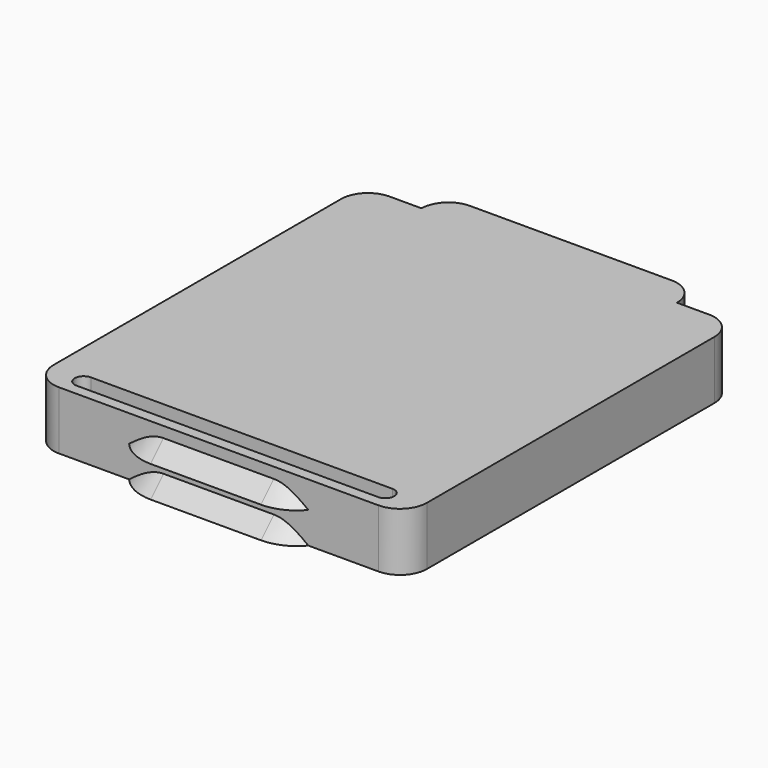
from build123d import *

# Parameters (mm, degrees)
F0_W        = 41.65
F0_H        = 46.1
F1_DEPTH    = 6.5
F2_W        = 28.5
F2_H        = 3
F3_DEPTH    = 3
F4_R        = 1
F5_T1_DEPTH = 10.5
F5_T4_ANGLE = 90
F5_T6_ANGLE = 90
F6_W        = 20
F6_H        = 1.8
F7_DEPTH    = 1.8
F8_T1_DEPTH = 21.0093727123
F8_T3_DEPTH = 21.0093727123
F9_SIZE2    = 1.79999
F9_SIZE     = 1.79999
F10_R       = 3


# Not quite as in the source:
# - a fillet or chamfer that OpenCascade refuses, or shapes differently, is made with other operations: its cross-section is extruded or revolved along the edge and cut away or added
# - a fillet or chamfer is up to 0.001 mm smaller than in the source, because OpenCascade refuses the exact size


with BuildPart() as f1:
    # F0 (on Top) → F1 (new body)
    with BuildSketch(Plane.XY):
        Rectangle(F0_W, F0_H)
        with BuildLine():
            ThreePointArc((16.825, -19.85), (17.825, -20.85), (16.825, -21.85))
            Line((16.825, -21.85), (-16.825, -21.85))
            ThreePointArc((-16.825, -21.85), (-17.825, -20.85), (-16.825, -19.85))
            Line((-16.825, -19.85), (16.825, -19.85))
        make_face(mode=Mode.SUBTRACT)
    extrude(amount=F1_DEPTH)

    # F2 (on face) → F3 (join)
    with BuildSketch(Plane(origin=(0, 23.05, 0), x_dir=(-1, 0, 0), z_dir=(0, 1, 0))):
        with Locations((0, 5)):
            Rectangle(F2_W, F2_H)
    extrude(amount=F3_DEPTH)

    # F4
    f4_edges = [f1.edges().sort_by_distance(p)[0] for p in [
        (-14.25, 24.55, 3.5),
        (14.25, 24.55, 3.5),
        (0, 26.05, 3.5),
    ]]
    fillet(f4_edges, radius=F4_R)

    # F5: fillet of radius 3 on 3 edges, made by hand

    # F5_s2 → F5_t1 (cut)
    with BuildSketch(Plane.XY.offset(3.5)):
        with BuildLine():
            ThreePointArc((14.25, 23.05), (13.3713203436, 25.1713203436), (11.25, 26.05))
            Line((11.25, 26.05), (14.25, 26.05))
            Line((14.25, 26.05), (14.25, 23.05))
        make_face()
        with BuildLine():
            ThreePointArc((-14.25, 23.05), (-13.3713203436, 25.1713203436), (-11.25, 26.05))
            Line((-11.25, 26.05), (-14.25, 26.05))
            Line((-14.25, 26.05), (-14.25, 23.05))
        make_face()
    extrude(amount=F5_T1_DEPTH, mode=Mode.SUBTRACT)

    # F5_s3 → F5_t4 (revolve, cut)
    with BuildSketch(Plane.XZ.offset(-23.05)):
        with BuildLine():
            ThreePointArc((-13.25, 3.5), (-13.9571067812, 3.7928932188), (-14.25, 4.5))
            Line((-14.25, 4.5), (-14.25, 3.5))
            Line((-14.25, 3.5), (-13.25, 3.5))
        make_face()
    revolve(axis=Axis((-11.25, 23.05, 3.5), (0, 0, -1)), revolution_arc=F5_T4_ANGLE, mode=Mode.SUBTRACT)

    # F5_s5 → F5_t6 (revolve, cut)
    with BuildSketch(Plane.YZ.offset(11.25)):
        with BuildLine():
            ThreePointArc((25.05, 3.5), (25.7571067812, 3.7928932188), (26.05, 4.5))
            Line((26.05, 4.5), (26.05, 3.5))
            Line((26.05, 3.5), (25.05, 3.5))
        make_face()
    revolve(axis=Axis((11.25, 23.05, 3.5), (0, 0, -1)), revolution_arc=F5_T6_ANGLE, mode=Mode.SUBTRACT)

    # F6 (on face) → F7 (join)
    with BuildSketch(Plane.XZ.offset(23.05)):
        with Locations((0, 4.4)):
            Rectangle(F6_W, F6_H)
        with Locations((0, 0.9)):
            Rectangle(F6_W, F6_H)
    extrude(amount=F7_DEPTH)

    # F8: fillet of radius 5 on 4 edges, made by hand

    # F8_s2 → F8_t1 (cut)
    with BuildSketch(Plane.XY.offset(-6.1046863561)):
        with BuildLine():
            ThreePointArc((-10, -23.05), (-8.2794458011, -24.3776925691), (-6.1581254575, -24.85))
            Line((-6.1581254575, -24.85), (-6.1581254575, -24.95))
            Line((-6.1581254575, -24.95), (-10, -24.95))
            Line((-10, -24.95), (-10.1, -24.85))
            ThreePointArc((-10.1, -24.85), (-10.1, -23.95), (-10.0768374908, -23.114))
            Line((-10.0768374908, -23.114), (-10, -23.05))
        make_face()
        with BuildLine():
            ThreePointArc((10, -23.05), (8.2794458011, -24.3776925691), (6.1581254575, -24.85))
            Line((6.1581254575, -24.85), (6.1581254575, -24.95))
            Line((6.1581254575, -24.95), (10, -24.95))
            Line((10, -24.95), (10.1, -24.85))
            ThreePointArc((10.1, -24.85), (10.1, -23.95), (10.0768374908, -23.114))
            Line((10.0768374908, -23.114), (10, -23.05))
        make_face()
    extrude(amount=F8_T1_DEPTH, mode=Mode.SUBTRACT)

    # F8_s4 → F8_t3 (cut)
    with BuildSketch(Plane.XY.offset(-9.6046863561)):
        with BuildLine():
            ThreePointArc((-10, -23.05), (-8.2794458011, -24.3776925691), (-6.1581254575, -24.85))
            Line((-6.1581254575, -24.85), (-6.1581254575, -24.95))
            Line((-6.1581254575, -24.95), (-10, -24.95))
            Line((-10, -24.95), (-10.1, -24.85))
            ThreePointArc((-10.1, -24.85), (-10.1, -23.95), (-10.0768374908, -23.114))
            Line((-10.0768374908, -23.114), (-10, -23.05))
        make_face()
        with BuildLine():
            ThreePointArc((10, -23.05), (8.2794458011, -24.3776925691), (6.1581254575, -24.85))
            Line((6.1581254575, -24.85), (6.1581254575, -24.95))
            Line((6.1581254575, -24.95), (10, -24.95))
            Line((10, -24.95), (10.1, -24.85))
            ThreePointArc((10.1, -24.85), (10.1, -23.95), (10.0768374908, -23.114))
            Line((10.0768374908, -23.114), (10, -23.05))
        make_face()
    extrude(amount=F8_T3_DEPTH, mode=Mode.SUBTRACT)

    # F9 (size 1.8 and 1.8 in the source; OpenCascade refuses exactly that, so slightly less here)
    f9_edges = [f1.edges().sort_by_distance(p)[0] for p in [
        (0, -24.85, 5.3),
        (0, -24.85, 1.8),
    ]]
    chamfer(f9_edges, length=F9_SIZE, length2=F9_SIZE2)

    # F10
    f10_edges = [f1.edges().sort_by_distance(p)[0] for p in [
        (20.825, -23.05, 3.25),
        (20.825, 23.05, 3.25),
        (-20.825, 23.05, 3.25),
        (-20.825, -23.05, 3.25),
    ]]
    fillet(f10_edges, radius=F10_R)


solid = f1.part
